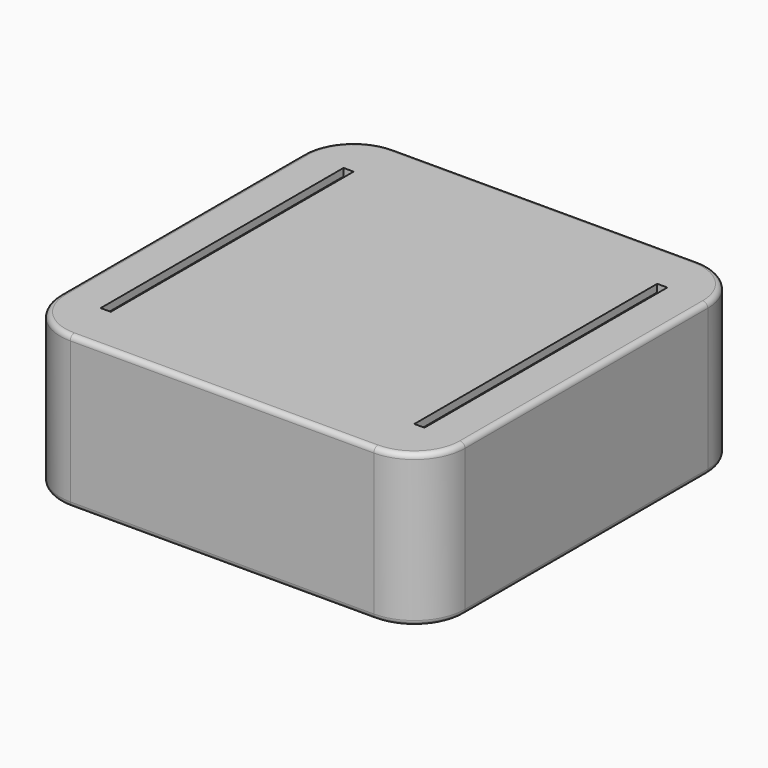
from build123d import *

# Parameters (mm, degrees)
F1_DEPTH    = 30
F2_T        = -1.5
F3_W        = 1.5
F3_H        = 4.25
F3_W_2      = 4.25
F3_H_2      = 1.5
F4_DEPTH    = 22
F5_SIZE     = 1.2
F6_R        = 1
F7_W        = 2
F7_H        = 60
F8_DEPTH    = 30.001
F10_SIZE2   = 2
F10_SIZE    = 5
F10_2_SIZE2 = 2
F10_2_SIZE  = 5
F10_3_SIZE2 = 2
F10_3_SIZE  = 5
F10_4_SIZE2 = 2
F10_4_SIZE  = 5
F10_5_SIZE2 = 2
F10_5_SIZE  = 5
F10_6_SIZE2 = 2
F10_6_SIZE  = 5
F10_7_SIZE2 = 2
F10_7_SIZE  = 5
F10_8_SIZE2 = 2
F10_8_SIZE  = 5


# Not quite as in the source:
# - a pattern or mirror of a feature is missing from the dataset's text; its kind, count and spacing are read off the source's solid


with BuildPart() as f1:
    # F0 (on Top) → F1 (new body)
    with BuildSketch(Plane.XY):
        with BuildLine():
            ThreePointArc((20, 10), (17.0710678119, 17.0710678119), (10, 20))
            Line((10, 20), (-50, 20))
            ThreePointArc((-50, 20), (-57.0710678119, 17.0710678119), (-60, 10))
            Line((-60, 10), (-60, -50))
            ThreePointArc((-60, -50), (-57.0710678119, -57.0710678119), (-50, -60))
            Line((-50, -60), (10, -60))
            ThreePointArc((10, -60), (17.0710678119, -57.0710678119), (20, -50))
            Line((20, -50), (20, 10))
        make_face()
    extrude(amount=F1_DEPTH)

    # F2
    f2_openings = [f1.faces().sort_by_distance(p)[0] for p in [
        (-20, -20, 0),
    ]]
    offset(amount=F2_T, openings=f2_openings)

    # F3 (on face) → F4 (join)
    with BuildSketch(Plane(origin=(0, 0, 28.5), x_dir=(1, 0, 0), z_dir=(0, 0, -1))):
        with Locations((-35.75, 56.375)):
            Rectangle(F3_W, F3_H)
        with Locations((-4.25, 56.375)):
            Rectangle(F3_W, F3_H)
        with Locations((-56.875, 4.25)):
            Rectangle(F3_W_2, F3_H_2)
        with Locations((-56.875, 35.75)):
            Rectangle(F3_W_2, F3_H_2)
        with Locations((-4.75, -16.875)):
            Rectangle(F3_W, F3_H)
        with Locations((-36.25, -16.875)):
            Rectangle(F3_W, F3_H)
        with Locations((16.375, 35.25)):
            Rectangle(F3_W_2, F3_H_2)
        with Locations((16.375, 3.75)):
            Rectangle(F3_W_2, F3_H_2)
    extrude(amount=F4_DEPTH)

    # F5
    f5_edges = [f1.edges().sort_by_distance(p)[0] for p in [
        (3, 18.5, 28.5),
        (-20.5, 18.5, 28.5),
        (-43.5, 18.5, 28.5),
        (18.5, -19.5, 28.5),
        (18.5, -43, 28.5),
        (-58.5, -20, 28.5),
        (-58.5, -43.25, 28.5),
        (-20, -58.5, 28.5),
        (16.010408, 16.010408, 28.5),
        (18.5, 3.5, 28.5),
        (16.010408, -56.010408, 28.5),
        (3.25, -58.5, 28.5),
        (-43.25, -58.5, 28.5),
        (-56.010408, -56.010408, 28.5),
        (-58.5, 3.25, 28.5),
        (-56.010408, 16.010408, 28.5),
    ]]
    chamfer(f5_edges, length=F5_SIZE)

    # F6
    f6_edges = [f1.edges().sort_by_distance(p)[0] for p in [
        (20, -20, 30),
        (20, -20, 0),
        (17.071068, 17.071068, 0),
        (-20, 20, 0),
        (-57.071068, 17.071068, 0),
        (-60, -20, 0),
        (-57.071068, -57.071068, 0),
        (-20, -60, 0),
        (17.071068, -57.071068, 0),
        (17.071068, 17.071068, 30),
        (-20, 20, 30),
        (-57.071068, 17.071068, 30),
        (-60, -20, 30),
        (-57.071068, -57.071068, 30),
        (-20, -60, 30),
        (17.071068, -57.071068, 30),
    ]]
    fillet(f6_edges, radius=F6_R)

    # F7 (on face) → F8 (cut, through all)
    with BuildSketch(Plane.XY.offset(30)):
        with Locations((-51, -20)):
            Rectangle(F7_W, F7_H)
    f8 = extrude(amount=-F8_DEPTH, mode=Mode.SUBTRACT)

    # F8_copies: F8 across plane
    add(f8.mirror(Plane(origin=(-20, 0, 0), x_dir=(0, 0, 1), z_dir=(1, 0, 0))), mode=Mode.SUBTRACT)

    # F10
    f10_edges = [f1.edges().sort_by_distance(p)[0] for p in [
        (-54.75, -4.25, 6.5),
    ]]
    f10_side = f1.faces().sort_by_distance((-54.75, -4.25, 17.5))[0]
    chamfer(f10_edges, length=F10_SIZE, length2=F10_SIZE2, reference=f10_side)

    # F10#2
    f10_2_edges = [f1.edges().sort_by_distance(p)[0] for p in [
        (-54.75, -35.75, 6.5),
    ]]
    f10_2_side = f1.faces().sort_by_distance((-54.75, -35.75, 17.5))[0]
    chamfer(f10_2_edges, length=F10_2_SIZE, length2=F10_2_SIZE2, reference=f10_2_side)

    # F10#3
    f10_3_edges = [f1.edges().sort_by_distance(p)[0] for p in [
        (-35.75, -54.25, 6.5),
    ]]
    f10_3_side = f1.faces().sort_by_distance((-35.75, -54.25, 17.5))[0]
    chamfer(f10_3_edges, length=F10_3_SIZE, length2=F10_3_SIZE2, reference=f10_3_side)

    # F10#4
    f10_4_edges = [f1.edges().sort_by_distance(p)[0] for p in [
        (-4.25, -54.25, 6.5),
    ]]
    f10_4_side = f1.faces().sort_by_distance((-4.25, -54.25, 17.5))[0]
    chamfer(f10_4_edges, length=F10_4_SIZE, length2=F10_4_SIZE2, reference=f10_4_side)

    # F10#5
    f10_5_edges = [f1.edges().sort_by_distance(p)[0] for p in [
        (14.25, -35.25, 6.5),
    ]]
    f10_5_side = f1.faces().sort_by_distance((14.25, -35.25, 17.5))[0]
    chamfer(f10_5_edges, length=F10_5_SIZE, length2=F10_5_SIZE2, reference=f10_5_side)

    # F10#6
    f10_6_edges = [f1.edges().sort_by_distance(p)[0] for p in [
        (14.25, -3.75, 6.5),
    ]]
    f10_6_side = f1.faces().sort_by_distance((14.25, -3.75, 17.5))[0]
    chamfer(f10_6_edges, length=F10_6_SIZE, length2=F10_6_SIZE2, reference=f10_6_side)

    # F10#7
    f10_7_edges = [f1.edges().sort_by_distance(p)[0] for p in [
        (-4.75, 14.75, 6.5),
    ]]
    f10_7_side = f1.faces().sort_by_distance((-4.75, 14.75, 17.5))[0]
    chamfer(f10_7_edges, length=F10_7_SIZE, length2=F10_7_SIZE2, reference=f10_7_side)

    # F10#8
    f10_8_edges = [f1.edges().sort_by_distance(p)[0] for p in [
        (-36.25, 14.75, 6.5),
    ]]
    f10_8_side = f1.faces().sort_by_distance((-36.25, 14.75, 17.5))[0]
    chamfer(f10_8_edges, length=F10_8_SIZE, length2=F10_8_SIZE2, reference=f10_8_side)


solid = f1.part
